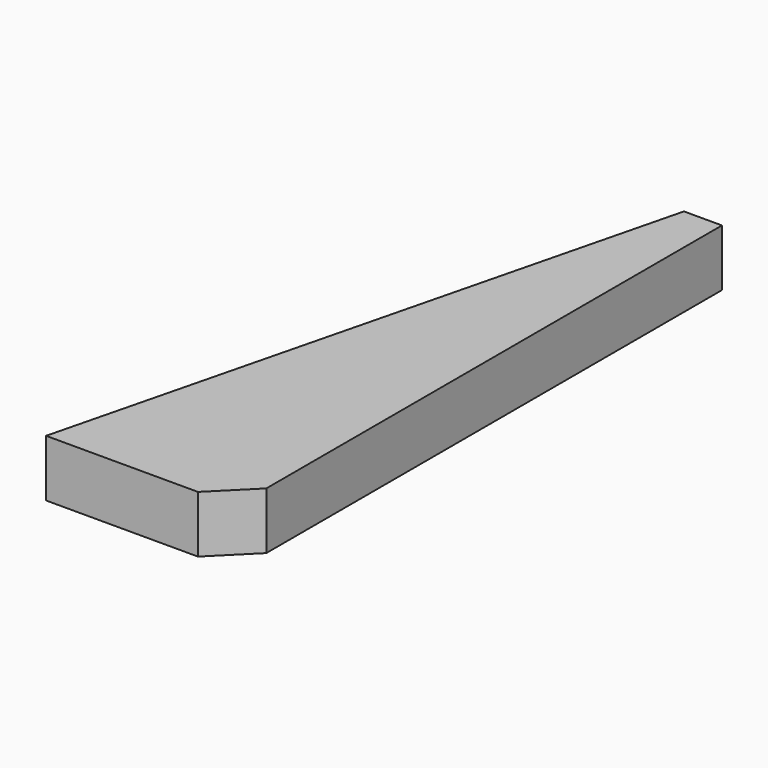
from build123d import *

# Parameters (mm, degrees)
F0_W     = 50
F0_H     = 160
F1_DEPTH = 15
F2_SIZE2 = 159.99999
F2_SIZE  = 39.99999
F3_SIZE2 = 10
F3_SIZE  = 10


# Not quite as in the source:
# - a fillet or chamfer is up to 0.001 mm smaller than in the source, because OpenCascade refuses the exact size


with BuildPart() as f1:
    # F0 (on Top) → F1 (new body)
    with BuildSketch(Plane.XY):
        Rectangle(F0_W, F0_H)
    extrude(amount=F1_DEPTH)

    # F2 (size 40 and 160 in the source; OpenCascade refuses exactly that, so slightly less here)
    f2_edges = [f1.edges().sort_by_distance(p)[0] for p in [
        (-25, 80, 7.5),
    ]]
    f2_side = f1.faces().sort_by_distance((0, 80, 7.5))[0]
    chamfer(f2_edges, length=F2_SIZE, length2=F2_SIZE2, reference=f2_side)

    # F3
    f3_edges = [f1.edges().sort_by_distance(p)[0] for p in [
        (25, -80, 7.5),
    ]]
    chamfer(f3_edges, length=F3_SIZE, length2=F3_SIZE2)


solid = f1.part
